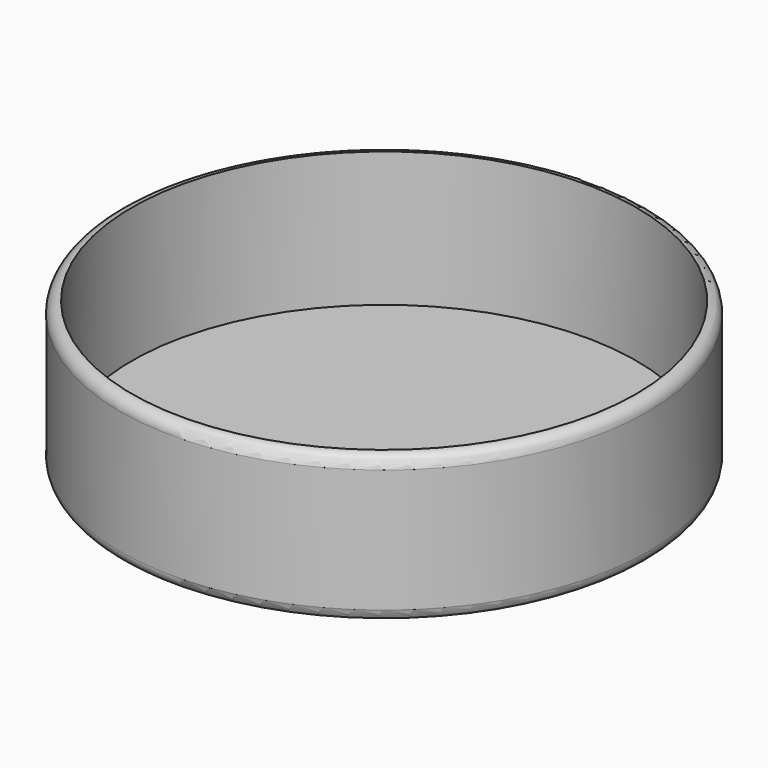
from build123d import *

# Parameters (mm, degrees)
F0_R     = 43
F1_DEPTH = 2
F0_R_2   = 45
F2_DEPTH = 25
F3_R     = 1.99999


# Not quite as in the source:
# - a fillet or chamfer is up to 0.001 mm smaller than in the source, because OpenCascade refuses the exact size


with BuildPart() as f1:
    # F0 (on Top) → F1 (new body)
    with BuildSketch(Plane.XY):
        Circle(F0_R)
    extrude(amount=F1_DEPTH)

    # F0 (on Top) → F2 (join)
    with BuildSketch(Plane.XY):
        Circle(F0_R_2)
        Circle(F0_R, mode=Mode.SUBTRACT)
    extrude(amount=F2_DEPTH)

    # F3 (radius 2 in the source; OpenCascade refuses exactly that, so slightly less here)
    f3_edges = [f1.edges().sort_by_distance(p)[0] for p in [
        (-45, 0, 0),
        (-45, 0, 25),
    ]]
    fillet(f3_edges, radius=F3_R)


solid = f1.part
